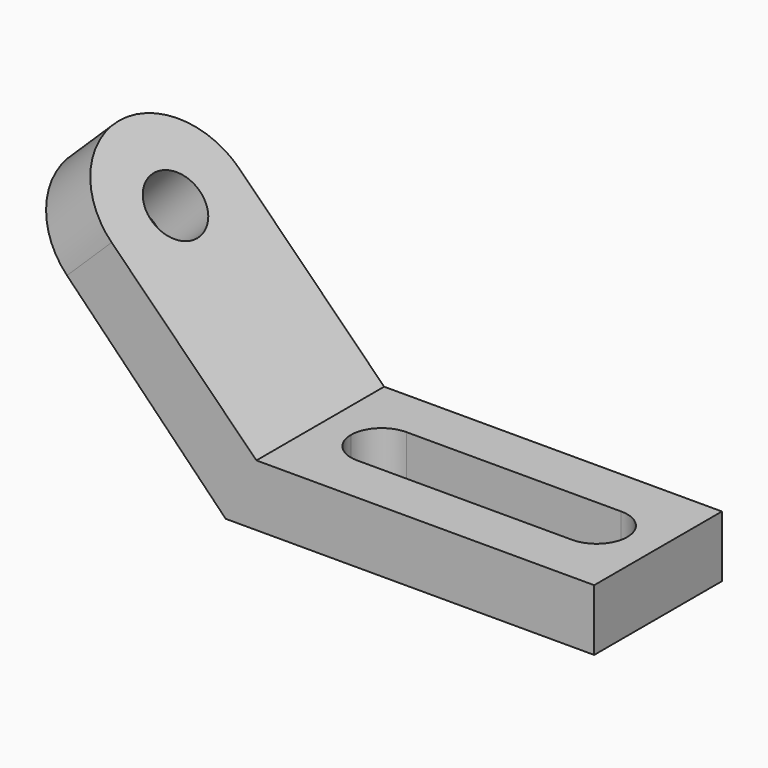
from build123d import *

# Parameters (mm, degrees)
F1_DEPTH = 52
F2_R     = 10
F3_DEPTH = 21
F5_DEPTH = 21
F6_R     = 25.99999


# Not quite as in the source:
# - a fillet or chamfer is up to 0.001 mm smaller than in the source, because OpenCascade refuses the exact size


with BuildPart() as f1:
    # F0 (on Front) → F1 (new body)
    with BuildSketch(Plane.XZ):
        Polygon((-69.8465537288, 71.5643691526), (0, 0), (120, 0), (120, 20), (10, 20), (-55.5336798983, 85.5336798983), align=None)
    extrude(amount=-F1_DEPTH)

    # F2 (on face) → F3 (cut)
    with BuildSketch(Plane(origin=(15, 0, 15), x_dir=(0.7071067812, 0, -0.7071067812), z_dir=(0.7071067812, 0, 0.7071067812))):
        with Locations((-73.7496867163, 26)):
            Circle(F2_R)
    extrude(amount=-F3_DEPTH, mode=Mode.SUBTRACT)

    # F4 (on face) → F5 (cut)
    with BuildSketch(Plane.XY.offset(20)):
        with BuildLine():
            ThreePointArc((20, 26), (22.9289321881, 18.9289321881), (30, 16))
            Line((30, 16), (100, 16))
            ThreePointArc((100, 16), (107.0710678119, 18.9289321881), (110, 26))
            ThreePointArc((110, 26), (107.0710678119, 33.0710678119), (100, 36))
            Line((100, 36), (30, 36))
            ThreePointArc((30, 36), (22.9289321881, 33.0710678119), (20, 26))
        make_face()
    extrude(amount=-F5_DEPTH, mode=Mode.SUBTRACT)

    # F6 (radius 26 in the source; OpenCascade refuses exactly that, so slightly less here)
    f6_edges = [f1.edges().sort_by_distance(p)[0] for p in [
        (-62.690117, 0, 78.549025),
        (-62.690117, 52, 78.549025),
    ]]
    fillet(f6_edges, radius=F6_R)


solid = f1.part
